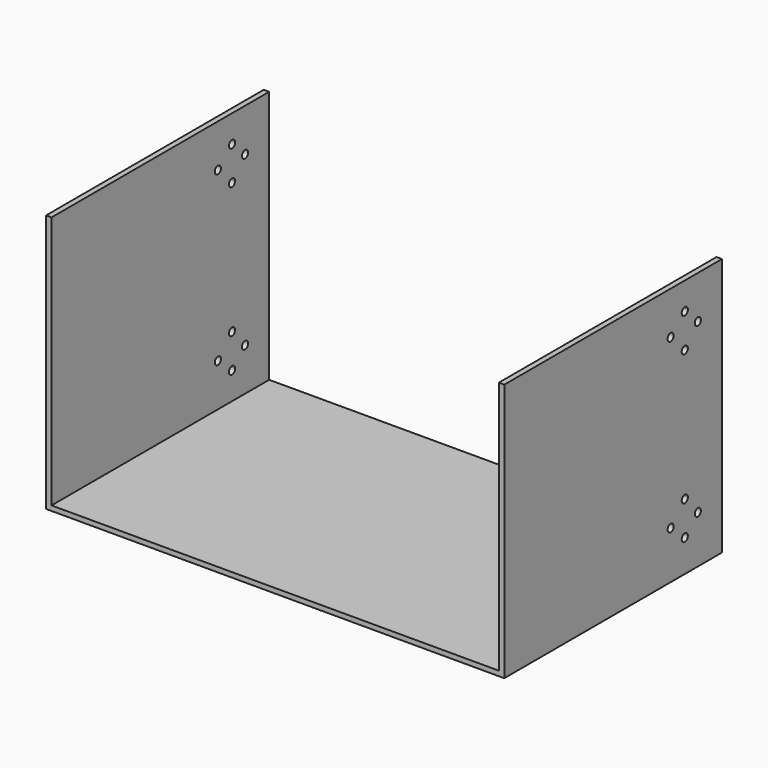
from build123d import *

# Parameters (mm, degrees)
F0_W     = 213.8947368421
F0_H     = 127
F1_DEPTH = 120.65
F2_W     = 208.8147368421
F2_H     = 127
F3_DEPTH = 118.364
F4_R     = 1.7907
F5_DEPTH = 220.472
F6_DEPTH = 25.4


# Not quite as in the source:
# - a pattern or mirror of a feature is missing from the dataset's text; its kind, count and spacing are read off the source's solid


with BuildPart() as f1:
    # F0 (on Top) → F1 (new body)
    with BuildSketch(Plane.XY):
        Rectangle(F0_W, F0_H)
    extrude(amount=F1_DEPTH)

    # F2 (on face) → F3 (cut)
    with BuildSketch(Plane.XY.offset(120.65)):
        Rectangle(F2_W, F2_H)
    extrude(amount=-F3_DEPTH, mode=Mode.SUBTRACT)

    # F4 (on face) → F5 (cut)
    with BuildSketch(Plane.YZ.offset(-104.4073684211)):
        with BuildLine():
            ThreePointArc((41.8333153324, 106.1593), (43.0995314454, 106.6837838869), (43.6240153324, 107.95))
            ThreePointArc((43.6240153324, 107.95), (40.5670992193, 109.2162161131), (41.8333153324, 106.1593))
        make_face()
        with BuildLine():
            ThreePointArc((51.2379409729, 100.683003664), (49.4472409729, 102.473703664), (47.6565409729, 100.683003664))
            ThreePointArc((47.6565409729, 100.683003664), (49.4472409729, 98.892303664), (51.2379409729, 100.683003664))
        make_face()
        with BuildLine():
            ThreePointArc((43.6240153324, 92.075), (43.0995314454, 93.3412161131), (41.8333153324, 93.8657))
            ThreePointArc((41.8333153324, 93.8657), (40.5670992193, 90.8087838869), (43.6240153324, 92.075))
        make_face()
        with Locations((33.5722409729, 100.683003664)):
            Circle(F4_R)
    f5 = extrude(amount=F5_DEPTH, mode=Mode.SUBTRACT)

    # F5_copies: F5 across plane
    add(f5.mirror(Plane(origin=(0, 0, 61.468), x_dir=(-1, 0, 0), z_dir=(0, 0, -1))), mode=Mode.SUBTRACT)

    # F4 (on face) → F6 (cut)
    with BuildSketch(Plane.YZ.offset(-104.4073684211)):
        with BuildLine():
            ThreePointArc((41.8333153324, 106.1593), (43.0995314454, 106.6837838869), (43.6240153324, 107.95))
            ThreePointArc((43.6240153324, 107.95), (40.5670992193, 109.2162161131), (41.8333153324, 106.1593))
        make_face()
        with BuildLine():
            ThreePointArc((51.2379409729, 100.683003664), (49.4472409729, 102.473703664), (47.6565409729, 100.683003664))
            ThreePointArc((47.6565409729, 100.683003664), (49.4472409729, 98.892303664), (51.2379409729, 100.683003664))
        make_face()
        with BuildLine():
            ThreePointArc((43.6240153324, 92.075), (43.0995314454, 93.3412161131), (41.8333153324, 93.8657))
            ThreePointArc((41.8333153324, 93.8657), (40.5670992193, 90.8087838869), (43.6240153324, 92.075))
        make_face()
        with Locations((33.5722409729, 100.683003664)):
            Circle(F4_R)
    f6 = extrude(amount=-F6_DEPTH, mode=Mode.SUBTRACT)

    # F6_copies: F6 across plane
    add(f6.mirror(Plane(origin=(0, 0, 61.468), x_dir=(-1, 0, 0), z_dir=(0, 0, -1))), mode=Mode.SUBTRACT)


solid = f1.part
